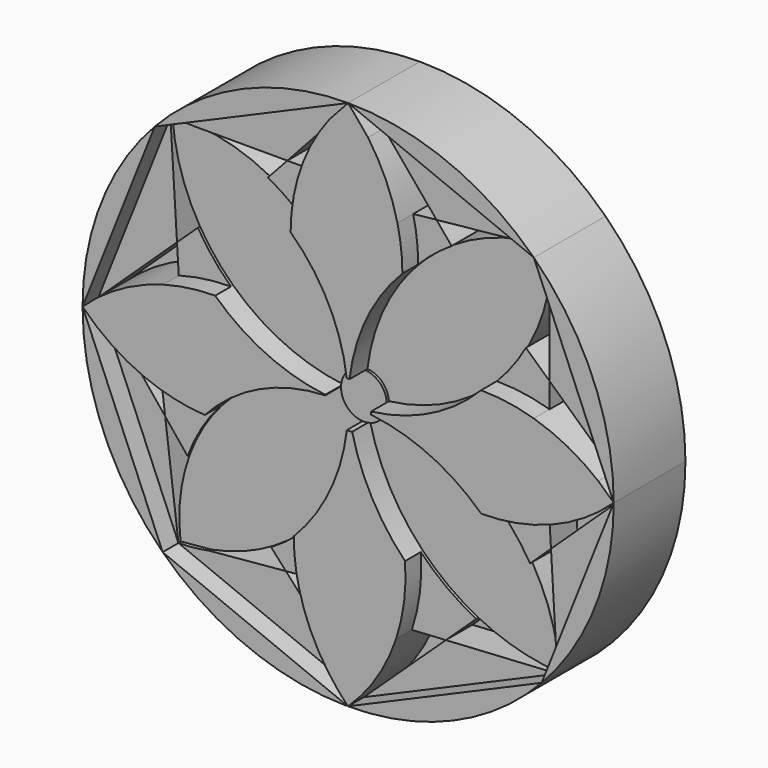
from build123d import *

# Parameters (mm, degrees)
F1_DEPTH = 25.4
F2_DEPTH = 19.05
F3_DEPTH = 19.812
F4_DEPTH = 10.414


# Not quite as in the source:
# - ends of sketch curves that miss each other by under 0.0002 mm in the source are joined


with BuildPart() as f1:
    # F0 (on Front) → F1 (new body)
    with BuildSketch(Plane.XZ):
        with BuildLine():
            Line((-75.2622127626, 0.0069578578), (-54.8323661222, 51.5539750531))
            ThreePointArc((-54.8323661222, 51.5539750531), (-69.9673038585, 27.7304365111), (-75.2622127626, 0.0069578578))
        make_face()
    extrude(amount=F1_DEPTH)


with BuildPart() as f1b:
    # F0 (on Front) → F1, piece 2 (new body)
    with BuildSketch(Plane.XZ):
        with BuildLine():
            Line((-54.8323661222, 51.5539750531), (0, 75.2622130842))
            ThreePointArc((0, 75.2622130842), (-29.8691685735, 69.08135412), (-54.8323661222, 51.5539750531))
        make_face()
    extrude(amount=F1_DEPTH)


with BuildPart() as f1c:
    # F0 (on Front) → F1, piece 3 (new body)
    with BuildSketch(Plane.XZ):
        with BuildLine():
            Line((0, 75.2622130842), (52.614982512, 53.8150939198))
            ThreePointArc((52.614982512, 53.8150939198), (28.4091327973, 69.694489682), (0, 75.2622130842))
        make_face()
    extrude(amount=F1_DEPTH)


with BuildPart() as f1d:
    # F0 (on Front) → F1, piece 4 (new body)
    with BuildSketch(Plane.XZ):
        with BuildLine():
            Line((52.614982512, 53.8150939198), (75.2622130842, 0))
            ThreePointArc((75.2622130842, 0), (69.3697367141, 29.1931558168), (52.614982512, 53.8150939198))
        make_face()
    extrude(amount=F1_DEPTH)


with BuildPart() as f1e:
    # F0 (on Front) → F1, piece 5 (new body)
    with BuildSketch(Plane.XZ):
        with BuildLine():
            ThreePointArc((54.8323661221, -51.5539750531), (69.9685855986, -27.7272023051), (75.2622130842, 0))
            Line((75.2622130842, 0), (54.8323661221, -51.5539750531))
        make_face()
    extrude(amount=F1_DEPTH)


with BuildPart() as f1f:
    # F0 (on Front) → F1, piece 6 (new body)
    with BuildSketch(Plane.XZ):
        with BuildLine():
            ThreePointArc((-0.0556531963, -75.2621925076), (29.8436251729, -69.0923928871), (54.8323661221, -51.5539750531))
            Line((54.8323661221, -51.5539750531), (-0.0556531963, -75.2621925076))
        make_face()
    extrude(amount=F1_DEPTH)


with BuildPart() as f1g:
    # F0 (on Front) → F1, piece 7 (new body)
    with BuildSketch(Plane.XZ):
        with BuildLine():
            ThreePointArc((-52.5567946174, -53.871922723), (-28.6128596995, -69.6110980961), (-0.5215979748, -75.2604056186))
            Line((-0.5215979748, -75.2604056186), (-0.6508580726, -75.0196912488))
            Line((-0.6508580726, -75.0196912488), (-52.5567946174, -53.871922723))
        make_face()
    extrude(amount=F1_DEPTH)


with BuildPart() as f1h:
    # F0 (on Front) → F1, piece 8 (new body)
    with BuildSketch(Plane.XZ):
        with BuildLine():
            Line((-52.5567946174, -53.871922723), (-75.2622127626, 0.0069578578))
            ThreePointArc((-75.2622127626, 0.0069578578), (-69.3553033665, -29.2274291252), (-52.5567946174, -53.871922723))
        make_face()
    extrude(amount=F1_DEPTH)


with BuildPart() as f1i:
    # F0 (on Front) → F1, piece 9 (new body)
    with BuildSketch(Plane.XZ):
        with BuildLine():
            ThreePointArc((-52.4700573047, 12.8987818425), (-64.6465144063, 7.8325449062), (-75.2622127626, 0.0069578578))
            ThreePointArc((-75.2622127626, 0.0069578578), (-67.1154289474, -6.8062849189), (-57.7657590343, -11.843549671))
            ThreePointArc((-57.7657590343, -11.843549671), (-49.3494805286, -14.5294310783), (-40.6023264953, -15.7683818996))
            ThreePointArc((-40.6023264953, -15.7683818996), (-25.1679784278, -4.3097622318), (-6.4822155283, 0.2025907933))
            ThreePointArc((-6.4822155283, 0.2025907933), (-6.478849637, 0.2909786351), (-6.4742785949, 0.3793123511))
            ThreePointArc((-6.4742785949, 0.3793123511), (-23.2491828543, 5.150765421), (-37.6813000828, 14.9425052875))
            ThreePointArc((-37.6813000828, 14.9425052875), (-45.1455174602, 14.4260096722), (-52.4700573047, 12.8987818425))
        make_face()
    extrude(amount=F1_DEPTH)


with BuildPart() as f1j:
    # F0 (on Front) → F1, piece 10 (new body)
    with BuildSketch(Plane.XZ):
        with BuildLine():
            ThreePointArc((52.5209722186, -12.8802052424), (64.6697465314, -7.8140081205), (75.2622130842, 0))
            Line((75.2622130842, 0), (70.8741968412, 4.0144167486))
            ThreePointArc((70.8741968412, 4.0144167486), (62.2236915492, 9.7505364956), (52.614982512, 13.6757144784))
            ThreePointArc((52.614982512, 13.6757144784), (45.2248075616, 15.3045595168), (37.6773561234, 15.8557389297))
            ThreePointArc((37.6773561234, 15.8557389297), (23.3925071535, 5.4667751122), (6.4733884939, 0.3942113542))
            ThreePointArc((6.4733884939, 0.3942113542), (6.4823818604, 0.1971968571), (6.4853805736, 0))
            ThreePointArc((6.4853805736, 0), (6.4827224307, -0.1856638671), (6.4747501808, -0.3711755392))
            ThreePointArc((6.4747501808, -0.3711755392), (23.2724799659, -5.1353425283), (37.7204536965, -14.9392737863))
            ThreePointArc((37.7204536965, -14.9392737863), (45.191142592, -14.4159854632), (52.5209722186, -12.8802052424))
        make_face()
    extrude(amount=F1_DEPTH)


with BuildPart() as f1k:
    # F0 (on Front) → F1, piece 11 (new body)
    with BuildSketch(Plane.XZ):
        with BuildLine():
            Line((5.6352679102, 68.4866793327), (0, 75.2622130842))
            Line((0, 75.2622130842), (-5.2994245304, 69.4754794646))
            ThreePointArc((-5.2994245304, 69.4754794646), (-10.7245630069, 60.961528287), (-14.3875446195, 51.5539750531))
            ThreePointArc((-14.3875446195, 51.5539750531), (-15.8147897939, 44.7040856548), (-16.3019121151, 37.7240623454))
            ThreePointArc((-16.3019121151, 37.7240623454), (-5.6093720428, 23.4928509105), (-0.3944758022, 6.4733723843))
            ThreePointArc((-0.3944758022, 6.4733723843), (-0.0072750916, 6.4853764931), (0.3799515761, 6.4742411126))
            ThreePointArc((0.3799515761, 6.4742411126), (5.2894832373, 23.3426466072), (15.377743482, 37.7257481607))
            ThreePointArc((15.377743482, 37.7257481607), (15.0186263549, 43.8337224623), (13.9674501619, 49.8612712006))
            ThreePointArc((13.9674501619, 49.8612712006), (10.6935675668, 59.5731098269), (5.6352679102, 68.4866793327))
        make_face()
    extrude(amount=F1_DEPTH)


with BuildPart() as f1l:
    # F0 (on Front) → F1, piece 12 (new body)
    with BuildSketch(Plane.XZ):
        with BuildLine():
            Line((-0.1911529806, -75.1129982272), (-0.0556531963, -75.2621925076))
            ThreePointArc((-0.0556531963, -75.2621925076), (8.0807409766, -65.4872348115), (13.5799608117, -54.0194848446))
            ThreePointArc((13.5799608117, -54.0194848446), (15.8587630573, -44.0244595464), (16.1173139126, -33.7762098498))
            ThreePointArc((16.1173139126, -33.7762098498), (6.7748947055, -21.0936437925), (1.1376129051, -6.3848256094))
            ThreePointArc((1.1376129051, -6.3848256094), (0.3849578429, -6.4739453692), (-0.3729547383, -6.4746479401))
            ThreePointArc((-0.3729547383, -6.4746479401), (-5.289816538, -23.4016872285), (-15.4198133688, -37.8267817945))
            ThreePointArc((-15.4198133688, -37.8267817945), (-15.0285599954, -44.1318751379), (-13.89952585, -50.3473850261))
            ThreePointArc((-13.89952585, -50.3473850261), (-9.6290122153, -61.9160508308), (-2.8318807644, -72.20538119))
            Line((-2.8318807644, -72.20538119), (-1.1932502666, -74.0096224231))
            Line((-1.1932502666, -74.0096224231), (-0.1911529806, -75.1129982272))
        make_face()
    extrude(amount=F1_DEPTH)


with BuildPart() as f2:
    # F0 (on Front) → F2 (new body)
    with BuildSketch(Plane.XZ):
        with BuildLine():
            Line((52.614982512, 51.3506147398), (52.614982512, 53.8150939198))
            Line((52.614982512, 53.8150939198), (43.9474458385, 52.9283645134))
            ThreePointArc((43.9474458385, 52.9283645134), (34.0299637846, 50.0843830014), (24.8388649788, 45.3973387438))
            ThreePointArc((24.8388649788, 45.3973387438), (19.8902154281, 41.8305052318), (15.377743482, 37.7257481607))
            ThreePointArc((15.377743482, 37.7257481607), (5.2894832373, 23.3426466072), (0.3799515761, 6.4742411126))
            ThreePointArc((0.3799515761, 6.4742411126), (4.5808032041, 4.5909043978), (6.4733884939, 0.3942113542))
            ThreePointArc((6.4733884939, 0.3942113542), (23.3925071535, 5.4667751122), (37.6773561234, 15.8557389297))
            ThreePointArc((37.6773561234, 15.8557389297), (42.1526303069, 21.0862424938), (45.9062846057, 26.8565393627))
            ThreePointArc((45.9062846057, 26.8565393627), (50.7615965469, 38.6924773424), (52.614982512, 51.3506147398))
        make_face()
    extrude(amount=F2_DEPTH)


with BuildPart() as f2b:
    # F0 (on Front) → F2, piece 2 (new body)
    with BuildSketch(Plane.XZ):
        with BuildLine():
            ThreePointArc((31.8487733101, -45.3540816238), (43.0232950327, -49.6301956737), (54.8323661221, -51.5539750531))
            ThreePointArc((54.8323661221, -51.5539750531), (52.4705239985, -38.5880027625), (47.08263839, -26.5603087055))
            ThreePointArc((47.08263839, -26.5603087055), (42.7987933835, -20.4297592527), (37.7204536965, -14.9392737863))
            ThreePointArc((37.7204536965, -14.9392737863), (23.2724799659, -5.1353425283), (6.4747501808, -0.3711755392))
            ThreePointArc((6.4747501808, -0.3711755392), (4.8505684955, -4.304897961), (1.1376129051, -6.3848256094))
            ThreePointArc((1.1376129051, -6.3848256094), (6.7748947055, -21.0936437925), (16.1173139126, -33.7762098498))
            ThreePointArc((16.1173139126, -33.7762098498), (23.4985623215, -40.2234357826), (31.8487733101, -45.3540816238))
        make_face()
    extrude(amount=F2_DEPTH)


with BuildPart() as f2c:
    # F0 (on Front) → F2, piece 3 (new body)
    with BuildSketch(Plane.XZ):
        with BuildLine():
            ThreePointArc((-15.4198133688, -37.8267817945), (-5.289816538, -23.4016872285), (-0.3729547383, -6.4746479401))
            ThreePointArc((-0.3729547383, -6.4746479401), (-4.7848426434, -4.377835317), (-6.4822155283, 0.2025907933))
            ThreePointArc((-6.4822155283, 0.2025907933), (-25.1679784278, -4.3097622318), (-40.6023264953, -15.7683818996))
            ThreePointArc((-40.6023264953, -15.7683818996), (-46.030453361, -23.1139216277), (-49.9748077084, -31.3518572883))
            ThreePointArc((-49.9748077084, -31.3518572883), (-52.6026172504, -42.4020706062), (-52.5704850767, -53.760396402))
            ThreePointArc((-52.5704850767, -53.760396402), (-52.5702860984, -53.762032881), (-52.5700870641, -53.7636693533))
            Line((-52.5700870641, -53.7636693533), (-43.8067720436, -52.9602114581))
            ThreePointArc((-43.8067720436, -52.9602114581), (-34.7670305391, -50.426749436), (-26.3062239068, -46.3585671123))
            ThreePointArc((-26.3062239068, -46.3585671123), (-20.5873469296, -42.4444267862), (-15.4198133688, -37.8267817945))
        make_face()
    extrude(amount=F2_DEPTH)


with BuildPart() as f2d:
    # F0 (on Front) → F2, piece 4 (new body)
    with BuildSketch(Plane.XZ):
        with BuildLine():
            Line((-48.2698807914, 51.5539750531), (-54.8323661222, 51.5539750531))
            ThreePointArc((-54.8323661222, 51.5539750531), (-52.4573293465, 38.5970695837), (-47.0643744392, 26.5788236053))
            ThreePointArc((-47.0643744392, 26.5788236053), (-42.7707081223, 20.4398368638), (-37.6813000828, 14.9425052875))
            ThreePointArc((-37.6813000828, 14.9425052875), (-23.2491828543, 5.150765421), (-6.4742785949, 0.3793123511))
            ThreePointArc((-6.4742785949, 0.3793123511), (-4.5912240921, 4.5804827825), (-0.3944758022, 6.4733723843))
            ThreePointArc((-0.3944758022, 6.4733723843), (-5.6093720428, 23.4928509105), (-16.3019121151, 37.7240623454))
            ThreePointArc((-16.3019121151, 37.7240623454), (-21.5001516409, 41.9936529211), (-27.2100841861, 45.5500230061))
            ThreePointArc((-27.2100841861, 45.5500230061), (-37.4174942383, 49.6831767785), (-48.2698807914, 51.5539750531))
        make_face()
    extrude(amount=F2_DEPTH)


with BuildPart() as f3:
    # F0 (on Front) → F3 (new body)
    with BuildSketch(Plane.XZ):
        with BuildLine():
            ThreePointArc((1.1376129051, -6.3848256094), (4.8505684955, -4.304897961), (6.4747501808, -0.3711755392))
            ThreePointArc((6.4747501808, -0.3711755392), (6.4827224307, -0.1856638671), (6.4853805736, 0))
            ThreePointArc((6.4853805736, 0), (6.4823818604, 0.1971968571), (6.4733884939, 0.3942113542))
            ThreePointArc((6.4733884939, 0.3942113542), (4.5808032041, 4.5909043978), (0.3799515761, 6.4742411126))
            ThreePointArc((0.3799515761, 6.4742411126), (-0.0072750916, 6.4853764931), (-0.3944758022, 6.4733723843))
            ThreePointArc((-0.3944758022, 6.4733723843), (-4.5912240921, 4.5804827825), (-6.4742785949, 0.3793123511))
            ThreePointArc((-6.4742785949, 0.3793123511), (-6.478849637, 0.2909786351), (-6.4822155283, 0.2025907933))
            ThreePointArc((-6.4822155283, 0.2025907933), (-4.7848426434, -4.377835317), (-0.3729547383, -6.4746479401))
            ThreePointArc((-0.3729547383, -6.4746479401), (0.3849578429, -6.4739453692), (1.1376129051, -6.3848256094))
        make_face()
    extrude(amount=F3_DEPTH)


with BuildPart() as f3b:
    # F0 (on Front) → F3, piece 2 (new body)
    with BuildSketch(Plane.XZ):
        Polygon((-52.9661997812, 21.0173153488), (-54.8323661222, 51.5539750531), (-75.2622127626, 0.0069578578), align=None)
    extrude(amount=F3_DEPTH)


with BuildPart() as f3c:
    # F0 (on Front) → F3, piece 3 (new body)
    with BuildSketch(Plane.XZ):
        with BuildLine():
            ThreePointArc((-5.2994245304, 69.4754794646), (-2.7599017928, 72.4697565848), (0, 75.2622130842))
            Line((0, 75.2622130842), (-54.8323661222, 51.5539750531))
            ThreePointArc((-54.8323661222, 51.5539750531), (-51.5511234568, 51.6585067903), (-48.2698807914, 51.5539750531))
            Line((-48.2698807914, 51.5539750531), (-21.7117335018, 51.5539750531))
            Line((-21.7117335018, 51.5539750531), (-5.2994245304, 69.4754794646))
        make_face()
    extrude(amount=F3_DEPTH)


with BuildPart() as f3d:
    # F0 (on Front) → F3, piece 4 (new body)
    with BuildSketch(Plane.XZ):
        with BuildLine():
            ThreePointArc((43.9474458385, 52.9283645134), (48.2632112907, 53.5477024744), (52.614982512, 53.8150939198))
            Line((52.614982512, 53.8150939198), (0, 75.2622130842))
            ThreePointArc((0, 75.2622130842), (2.9567761175, 71.990171905), (5.6352679102, 68.4866793327))
            Line((5.6352679102, 68.4866793327), (20.5648204682, 50.5362129373))
            Line((20.5648204682, 50.5362129373), (43.9474458385, 52.9283645134))
        make_face()
    extrude(amount=F3_DEPTH)


with BuildPart() as f3e:
    # F0 (on Front) → F3, piece 5 (new body)
    with BuildSketch(Plane.XZ):
        with BuildLine():
            ThreePointArc((70.8741968412, 4.0144167486), (73.1250050308, 2.0692945097), (75.2622130842, 0))
            Line((75.2622130842, 0), (52.614982512, 53.8150939198))
            ThreePointArc((52.614982512, 53.8150939198), (52.6294227925, 52.5828543298), (52.614982512, 51.3506147398))
            Line((52.614982512, 51.3506147398), (52.614982512, 20.7190257929))
            Line((52.614982512, 20.7190257929), (70.8741968412, 4.0144167486))
        make_face()
    extrude(amount=F3_DEPTH)


with BuildPart() as f3f:
    # F0 (on Front) → F3, piece 6 (new body)
    with BuildSketch(Plane.XZ):
        Polygon((54.8323661221, -51.5539750531), (75.2622130842, 0), (53.0049661188, -20.9782921406), align=None)
    extrude(amount=F3_DEPTH)


with BuildPart() as f3g:
    # F0 (on Front) → F3, piece 7 (new body)
    with BuildSketch(Plane.XZ):
        Polygon((-0.0556531963, -75.2621925076), (54.8323661221, -51.5539750531), (23.2195483504, -53.4433609244), align=None)
    extrude(amount=F3_DEPTH)


with BuildPart() as f3h:
    # F0 (on Front) → F3, piece 8 (new body)
    with BuildSketch(Plane.XZ):
        with BuildLine():
            Line((-52.5567946174, -53.871922723), (-0.6508580726, -75.0196912488))
            Line((-0.6508580726, -75.0196912488), (-1.1206071389, -74.1449019487))
            ThreePointArc((-1.1206071389, -74.1449019487), (-1.9879238823, -73.1854469797), (-2.8318807644, -72.20538119))
            Line((-2.8318807644, -72.20538119), (-22.1166519237, -50.9715646926))
            Line((-22.1166519237, -50.9715646926), (-43.8067720436, -52.9602114581))
            ThreePointArc((-43.8067720436, -52.9602114581), (-48.163092884, -53.5954460617), (-52.5567946174, -53.871922723))
        make_face()
    extrude(amount=F3_DEPTH)


with BuildPart() as f3i:
    # F0 (on Front) → F3, piece 9 (new body)
    with BuildSketch(Plane.XZ):
        with BuildLine():
            Line((-56.3237204559, -23.4785946581), (-75.2622127626, 0.0069578578))
            Line((-75.2622127626, 0.0069578578), (-52.5567946174, -53.871922723))
            ThreePointArc((-52.5567946174, -53.871922723), (-52.5634714728, -53.8177997995), (-52.5700870641, -53.7636693533))
            Line((-52.5700870641, -53.7636693533), (-52.5879003108, -53.7653043866))
            Line((-52.5879003108, -53.7653043866), (-52.5706126484, -53.7604323544))
            Line((-52.5706126484, -53.7604323544), (-56.3237204559, -23.4785946581))
        make_face()
    extrude(amount=F3_DEPTH)


with BuildPart() as f3j:
    # F0 (on Front) → F3, piece 10 (new body)
    with BuildSketch(Plane.XZ):
        with BuildLine():
            ThreePointArc((-40.6023264953, -15.7683818996), (-49.3494805286, -14.5294310783), (-57.7657590343, -11.843549671))
            Line((-57.7657590343, -11.843549671), (-56.3237204559, -23.4785946581))
            Line((-56.3237204559, -23.4785946581), (-49.9748077084, -31.3518572883))
            ThreePointArc((-49.9748077084, -31.3518572883), (-46.030453361, -23.1139216277), (-40.6023264953, -15.7683818996))
        make_face()
    extrude(amount=F3_DEPTH)


with BuildPart() as f3k:
    # F0 (on Front) → F3, piece 11 (new body)
    with BuildSketch(Plane.XZ):
        with BuildLine():
            Line((-26.3062239068, -46.3585671123), (-22.1166519237, -50.9715646926))
            Line((-22.1166519237, -50.9715646926), (-13.9656504616, -50.2242445946))
            Line((-13.9656504616, -50.2242445946), (-13.89952585, -50.3473850261))
            ThreePointArc((-13.89952585, -50.3473850261), (-15.0285599954, -44.1318751379), (-15.4198133688, -37.8267817945))
            ThreePointArc((-15.4198133688, -37.8267817945), (-20.5873469296, -42.4444267862), (-26.3062239068, -46.3585671123))
        make_face()
    extrude(amount=F3_DEPTH)


with BuildPart() as f3l:
    # F0 (on Front) → F3, piece 12 (new body)
    with BuildSketch(Plane.XZ):
        with BuildLine():
            Line((23.2195483504, -53.4433609244), (31.8487733101, -45.3540816238))
            ThreePointArc((31.8487733101, -45.3540816238), (23.4985623215, -40.2234357826), (16.1173139126, -33.7762098498))
            ThreePointArc((16.1173139126, -33.7762098498), (15.8587630573, -44.0244595464), (13.5799608117, -54.0194848446))
            Line((13.5799608117, -54.0194848446), (23.2195483504, -53.4433609244))
        make_face()
    extrude(amount=F3_DEPTH)


with BuildPart() as f3m:
    # F0 (on Front) → F3, piece 13 (new body)
    with BuildSketch(Plane.XZ):
        with BuildLine():
            Line((53.0049661188, -20.9782921406), (52.5209722186, -12.8802052424))
            ThreePointArc((52.5209722186, -12.8802052424), (45.191142592, -14.4159854632), (37.7204536965, -14.9392737863))
            ThreePointArc((37.7204536965, -14.9392737863), (42.7987933835, -20.4297592527), (47.08263839, -26.5603087055))
            Line((47.08263839, -26.5603087055), (53.0049661188, -20.9782921406))
        make_face()
    extrude(amount=F3_DEPTH)


with BuildPart() as f3n:
    # F0 (on Front) → F3, piece 14 (new body)
    with BuildSketch(Plane.XZ):
        with BuildLine():
            ThreePointArc((37.6773561234, 15.8557389297), (45.2248075616, 15.3045595168), (52.614982512, 13.6757144784))
            Line((52.614982512, 13.6757144784), (52.614982512, 20.7190257929))
            Line((52.614982512, 20.7190257929), (45.9062846057, 26.8565393627))
            ThreePointArc((45.9062846057, 26.8565393627), (42.1526303069, 21.0862424938), (37.6773561234, 15.8557389297))
        make_face()
    extrude(amount=F3_DEPTH)


with BuildPart() as f3o:
    # F0 (on Front) → F3, piece 15 (new body)
    with BuildSketch(Plane.XZ):
        with BuildLine():
            ThreePointArc((15.377743482, 37.7257481607), (19.8902154281, 41.8305052318), (24.8388649788, 45.3973387438))
            Line((24.8388649788, 45.3973387438), (20.5648204682, 50.5362129373))
            Line((20.5648204682, 50.5362129373), (13.9674501619, 49.8612712006))
            ThreePointArc((13.9674501619, 49.8612712006), (15.0186263549, 43.8337224623), (15.377743482, 37.7257481607))
        make_face()
    extrude(amount=F3_DEPTH)


with BuildPart() as f3p:
    # F0 (on Front) → F3, piece 16 (new body)
    with BuildSketch(Plane.XZ):
        with BuildLine():
            ThreePointArc((-16.3019121151, 37.7240623454), (-15.8147897939, 44.7040856548), (-14.3875446195, 51.5539750531))
            Line((-14.3875446195, 51.5539750531), (-21.7117335018, 51.5539750531))
            Line((-21.7117335018, 51.5539750531), (-27.2100841861, 45.5500230061))
            ThreePointArc((-27.2100841861, 45.5500230061), (-21.5001516409, 41.9936529211), (-16.3019121151, 37.7240623454))
        make_face()
    extrude(amount=F3_DEPTH)


with BuildPart() as f3q:
    # F0 (on Front) → F3, piece 17 (new body)
    with BuildSketch(Plane.XZ):
        with BuildLine():
            ThreePointArc((-37.6813000828, 14.9425052875), (-42.7707081223, 20.4398368638), (-47.0643744392, 26.5788236053))
            Line((-47.0643744392, 26.5788236053), (-52.9661997812, 21.0173153488))
            Line((-52.9661997812, 21.0173153488), (-52.4700573047, 12.8987818425))
            ThreePointArc((-52.4700573047, 12.8987818425), (-45.1455174602, 14.4260096722), (-37.6813000828, 14.9425052875))
        make_face()
    extrude(amount=F3_DEPTH)


with BuildPart() as f4:
    # F0 (on Front) → F4 (new body)
    with BuildSketch(Plane.XZ):
        with BuildLine():
            Line((20.5648204682, 50.5362129373), (5.6352679102, 68.4866793327))
            ThreePointArc((5.6352679102, 68.4866793327), (10.6935675668, 59.5731098269), (13.9674501619, 49.8612712006))
            Line((13.9674501619, 49.8612712006), (20.5648204682, 50.5362129373))
        make_face()
    extrude(amount=F4_DEPTH)


with BuildPart() as f4b:
    # F0 (on Front) → F4, piece 2 (new body)
    with BuildSketch(Plane.XZ):
        with BuildLine():
            ThreePointArc((24.8388649788, 45.3973387438), (34.0299637846, 50.0843830014), (43.9474458385, 52.9283645134))
            Line((43.9474458385, 52.9283645134), (20.5648204682, 50.5362129373))
            Line((20.5648204682, 50.5362129373), (24.8388649788, 45.3973387438))
        make_face()
    extrude(amount=F4_DEPTH)


with BuildPart() as f4c:
    # F0 (on Front) → F4, piece 3 (new body)
    with BuildSketch(Plane.XZ):
        with BuildLine():
            Line((52.614982512, 20.7190257929), (52.614982512, 51.3506147398))
            ThreePointArc((52.614982512, 51.3506147398), (50.7615965469, 38.6924773424), (45.9062846057, 26.8565393627))
            Line((45.9062846057, 26.8565393627), (52.614982512, 20.7190257929))
        make_face()
    extrude(amount=F4_DEPTH)


with BuildPart() as f4d:
    # F0 (on Front) → F4, piece 4 (new body)
    with BuildSketch(Plane.XZ):
        with BuildLine():
            ThreePointArc((52.614982512, 13.6757144784), (62.2236915492, 9.7505364956), (70.8741968412, 4.0144167486))
            Line((70.8741968412, 4.0144167486), (52.614982512, 20.7190257929))
            Line((52.614982512, 20.7190257929), (52.614982512, 13.6757144784))
        make_face()
    extrude(amount=F4_DEPTH)


with BuildPart() as f4e:
    # F0 (on Front) → F4, piece 5 (new body)
    with BuildSketch(Plane.XZ):
        with BuildLine():
            Line((53.0049661188, -20.9782921406), (75.2622130842, 0))
            ThreePointArc((75.2622130842, 0), (64.6697465314, -7.8140081205), (52.5209722186, -12.8802052424))
            Line((52.5209722186, -12.8802052424), (53.0049661188, -20.9782921406))
        make_face()
    extrude(amount=F4_DEPTH)


with BuildPart() as f4f:
    # F0 (on Front) → F4, piece 6 (new body)
    with BuildSketch(Plane.XZ):
        with BuildLine():
            ThreePointArc((47.08263839, -26.5603087055), (52.4705239985, -38.5880027625), (54.8323661221, -51.5539750531))
            Line((54.8323661221, -51.5539750531), (53.0049661188, -20.9782921406))
            Line((53.0049661188, -20.9782921406), (47.08263839, -26.5603087055))
        make_face()
    extrude(amount=F4_DEPTH)


with BuildPart() as f4g:
    # F0 (on Front) → F4, piece 7 (new body)
    with BuildSketch(Plane.XZ):
        with BuildLine():
            Line((23.2195483504, -53.4433609244), (54.8323661221, -51.5539750531))
            ThreePointArc((54.8323661221, -51.5539750531), (43.0232950327, -49.6301956737), (31.8487733101, -45.3540816238))
            Line((31.8487733101, -45.3540816238), (23.2195483504, -53.4433609244))
        make_face()
    extrude(amount=F4_DEPTH)


with BuildPart() as f4h:
    # F0 (on Front) → F4, piece 8 (new body)
    with BuildSketch(Plane.XZ):
        with BuildLine():
            ThreePointArc((13.5799608117, -54.0194848446), (8.0807409766, -65.4872348115), (-0.0556531963, -75.2621925076))
            Line((-0.0556531963, -75.2621925076), (23.2195483504, -53.4433609244))
            Line((23.2195483504, -53.4433609244), (13.5799608117, -54.0194848446))
        make_face()
    extrude(amount=F4_DEPTH)


with BuildPart() as f4i:
    # F0 (on Front) → F4, piece 9 (new body)
    with BuildSketch(Plane.XZ):
        with BuildLine():
            Line((-22.1166519237, -50.9715646926), (-2.8318807644, -72.20538119))
            ThreePointArc((-2.8318807644, -72.20538119), (-9.6290122153, -61.9160508308), (-13.89952585, -50.3473850261))
            Line((-13.89952585, -50.3473850261), (-13.9656504616, -50.2242445946))
            Line((-13.9656504616, -50.2242445946), (-22.1166519237, -50.9715646926))
        make_face()
    extrude(amount=F4_DEPTH)


with BuildPart() as f4j:
    # F0 (on Front) → F4, piece 10 (new body)
    with BuildSketch(Plane.XZ):
        with BuildLine():
            ThreePointArc((-26.3062239068, -46.3585671123), (-34.7670305391, -50.426749436), (-43.8067720436, -52.9602114581))
            Line((-43.8067720436, -52.9602114581), (-22.1166519237, -50.9715646926))
            Line((-22.1166519237, -50.9715646926), (-26.3062239068, -46.3585671123))
        make_face()
    extrude(amount=F4_DEPTH)


with BuildPart() as f4k:
    # F0 (on Front) → F4, piece 11 (new body)
    with BuildSketch(Plane.XZ):
        with BuildLine():
            Line((-49.9748077084, -31.3518572883), (-56.3237204559, -23.4785946581))
            Line((-56.3237204559, -23.4785946581), (-52.5706126484, -53.7604323544))
            Line((-52.5706126484, -53.7604323544), (-52.5704850767, -53.760396402))
            ThreePointArc((-52.5704850767, -53.760396402), (-52.6026172504, -42.4020706062), (-49.9748077084, -31.3518572883))
        make_face()
    extrude(amount=F4_DEPTH)


with BuildPart() as f4l:
    # F0 (on Front) → F4, piece 12 (new body)
    with BuildSketch(Plane.XZ):
        with BuildLine():
            ThreePointArc((-57.7657590343, -11.843549671), (-67.1154289474, -6.8062849189), (-75.2622127626, 0.0069578578))
            Line((-75.2622127626, 0.0069578578), (-56.3237204559, -23.4785946581))
            Line((-56.3237204559, -23.4785946581), (-57.7657590343, -11.843549671))
        make_face()
    extrude(amount=F4_DEPTH)


with BuildPart() as f4m:
    # F0 (on Front) → F4, piece 13 (new body)
    with BuildSketch(Plane.XZ):
        with BuildLine():
            Line((-52.9661997812, 21.0173153488), (-75.2622127626, 0.0069578578))
            ThreePointArc((-75.2622127626, 0.0069578578), (-64.6465144063, 7.8325449062), (-52.4700573047, 12.8987818425))
            Line((-52.4700573047, 12.8987818425), (-52.9661997812, 21.0173153488))
        make_face()
    extrude(amount=F4_DEPTH)


with BuildPart() as f4n:
    # F0 (on Front) → F4, piece 14 (new body)
    with BuildSketch(Plane.XZ):
        with BuildLine():
            ThreePointArc((-47.0643744392, 26.5788236053), (-52.4573293465, 38.5970695837), (-54.8323661222, 51.5539750531))
            Line((-54.8323661222, 51.5539750531), (-52.9661997812, 21.0173153488))
            Line((-52.9661997812, 21.0173153488), (-47.0643744392, 26.5788236053))
        make_face()
    extrude(amount=F4_DEPTH)


with BuildPart() as f4o:
    # F0 (on Front) → F4, piece 15 (new body)
    with BuildSketch(Plane.XZ):
        with BuildLine():
            Line((-21.7117335018, 51.5539750531), (-48.2698807914, 51.5539750531))
            ThreePointArc((-48.2698807914, 51.5539750531), (-37.4174942383, 49.6831767785), (-27.2100841861, 45.5500230061))
            Line((-27.2100841861, 45.5500230061), (-21.7117335018, 51.5539750531))
        make_face()
    extrude(amount=F4_DEPTH)


with BuildPart() as f4p:
    # F0 (on Front) → F4, piece 16 (new body)
    with BuildSketch(Plane.XZ):
        with BuildLine():
            ThreePointArc((-14.3875446195, 51.5539750531), (-10.7245630069, 60.961528287), (-5.2994245304, 69.4754794646))
            Line((-5.2994245304, 69.4754794646), (-21.7117335018, 51.5539750531))
            Line((-21.7117335018, 51.5539750531), (-14.3875446195, 51.5539750531))
        make_face()
    extrude(amount=F4_DEPTH)


solid = Compound([f1.part, f1b.part, f1c.part, f1d.part, f1e.part, f1f.part, f1g.part, f1h.part, f1i.part, f1j.part, f1k.part, f1l.part, f2.part, f2b.part, f2c.part, f2d.part, f3.part, f3b.part, f3c.part, f3d.part, f3e.part, f3f.part, f3g.part, f3h.part, f3i.part, f3j.part, f3k.part, f3l.part, f3m.part, f3n.part, f3o.part, f3p.part, f3q.part, f4.part, f4b.part, f4c.part, f4d.part, f4e.part, f4f.part, f4g.part, f4h.part, f4i.part, f4j.part, f4k.part, f4l.part, f4m.part, f4n.part, f4o.part, f4p.part])
